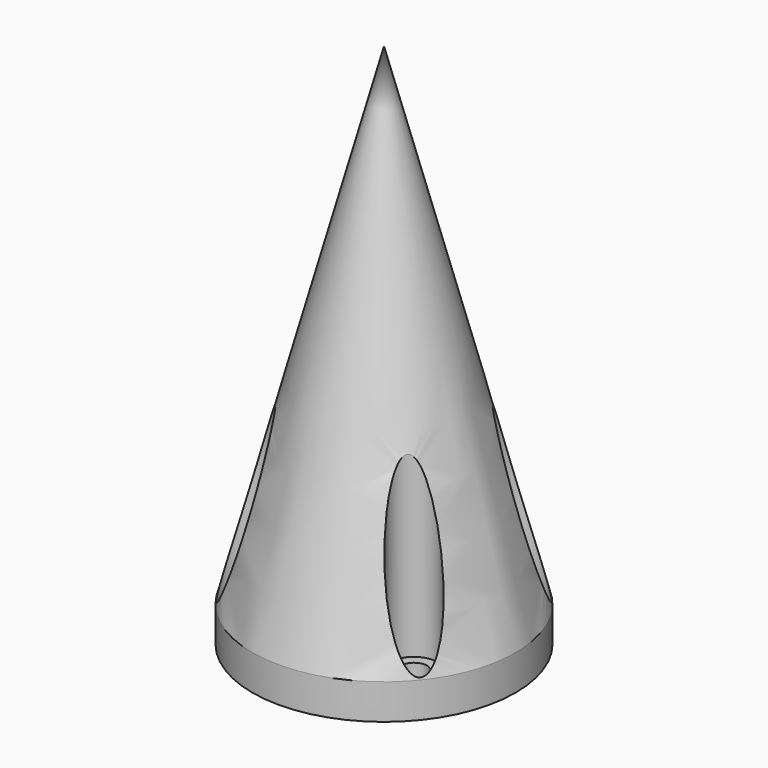
from build123d import *

# Parameters (mm, degrees)
F0_R           = 1.25
F1_DEPTH       = 5
F3_D           = 2.5
F3_DEPTH       = 5
F3_CBORE_D     = 4.4
F3_CBORE_DEPTH = 2
F3_TIP         = 0.7510757738
F4_DEPTH       = 45


# Not quite as in the source:
# - a fillet or chamfer that OpenCascade refuses, or shapes differently, is made with other operations: its cross-section is extruded or revolved along the edge and cut away or added


with BuildPart() as f1:
    # F0 (on Top) → F1 (new body)
    with BuildSketch(Plane.XY):
        with BuildLine():
            ThreePointArc((9.7397717911, -7.8349757789), (11.7897656336, -4.1534836349), (12.5, 0))
            ThreePointArc((12.5, 0), (11.7897656358, 4.1534836287), (9.7397717994, 7.8349757687))
            ThreePointArc((9.7397717994, 7.8349757687), (6.6e-09, 12.5), (-9.7397717911, 7.8349757789))
            ThreePointArc((-9.7397717911, 7.8349757789), (-12.5, 0), (-9.7397717911, -7.8349757789))
            ThreePointArc((-9.7397717911, -7.8349757789), (0, -12.5), (9.7397717911, -7.8349757789))
        make_face()
        with BuildLine():
            ThreePointArc((-5.7366128015, -6.4246802223), (-7.2389857978, -8.5468380541), (-9.7397717911, -7.8349757789))
            ThreePointArc((-9.7397717911, -7.8349757789), (-8.7342398052, -4.3025223904), (-5.7366128015, -6.4246802223))
        make_face(mode=Mode.SUBTRACT)
        with BuildLine():
            ThreePointArc((10.2366128015, -6.4246802223), (10.1087706334, -7.172307226), (9.7397717911, -7.8349757789))
            ThreePointArc((9.7397717911, -7.8349757789), (5.8644549697, -5.6770532186), (10.2366128015, -6.4246802223))
        make_face(mode=Mode.SUBTRACT)
        with BuildLine():
            ThreePointArc((-5.7366128015, 6.4246802223), (-8.7342398052, 4.3025223904), (-9.7397717911, 7.8349757789))
            ThreePointArc((-9.7397717911, 7.8349757789), (-7.2389857978, 8.5468380541), (-5.7366128015, 6.4246802223))
        make_face(mode=Mode.SUBTRACT)
        with BuildLine():
            ThreePointArc((10.2366128015, 6.4246802223), (5.8644549675, 5.6770532248), (9.7397717994, 7.8349757687))
            ThreePointArc((9.7397717994, 7.8349757687), (10.1087706356, 7.1723072198), (10.2366128015, 6.4246802223))
        make_face(mode=Mode.SUBTRACT)
        with BuildLine():
            ThreePointArc((10.2366128015, 6.4246802223), (10.1087706356, 7.1723072198), (9.7397717994, 7.8349757687))
            ThreePointArc((9.7397717994, 7.8349757687), (5.8644549675, 5.6770532248), (10.2366128015, 6.4246802223))
        make_face()
        with Locations((7.9866128015, 6.4246802223)):
            Circle(F0_R, mode=Mode.SUBTRACT)
        with BuildLine():
            ThreePointArc((10.2366128015, -6.4246802223), (5.8644549697, -5.6770532186), (9.7397717911, -7.8349757789))
            ThreePointArc((9.7397717911, -7.8349757789), (10.1087706334, -7.172307226), (10.2366128015, -6.4246802223))
        make_face()
        with Locations((7.9866128015, -6.4246802223)):
            Circle(F0_R, mode=Mode.SUBTRACT)
        with BuildLine():
            ThreePointArc((-5.7366128015, -6.4246802223), (-8.7342398052, -4.3025223904), (-9.7397717911, -7.8349757789))
            ThreePointArc((-9.7397717911, -7.8349757789), (-7.2389857978, -8.5468380541), (-5.7366128015, -6.4246802223))
        make_face()
        with Locations((-7.9866128015, -6.4246802223)):
            Circle(F0_R, mode=Mode.SUBTRACT)
        with BuildLine():
            ThreePointArc((-5.7366128015, 6.4246802223), (-7.2389857978, 8.5468380541), (-9.7397717911, 7.8349757789))
            ThreePointArc((-9.7397717911, 7.8349757789), (-8.7342398052, 4.3025223904), (-5.7366128015, 6.4246802223))
        make_face()
        with Locations((-7.9866128015, 6.4246802223)):
            Circle(F0_R, mode=Mode.SUBTRACT)
        with Locations((7.9866128015, 6.4246802223)):
            Circle(F0_R)
        with Locations((7.9866128015, -6.4246802223)):
            Circle(F0_R)
        with Locations((-7.9866128015, -6.4246802223)):
            Circle(F0_R)
        with Locations((-7.9866128015, 6.4246802223)):
            Circle(F0_R)
    extrude(amount=F1_DEPTH)

    # F3
    with Locations(Plane.XY.offset(5)):
        with Locations((-7.9866128015, 6.4246802223), (-7.9866128015, -6.4246802223), (7.9866128015, -6.4246802223), (7.9866128015, 6.4246802223)):
            CounterBoreHole(F3_D / 2, F3_CBORE_D / 2, F3_CBORE_DEPTH, depth=F3_DEPTH)
            with Locations((0, 0, -(F3_DEPTH + F3_TIP / 2))):  # 118° drill point
                Cone(0, F3_D / 2, F3_TIP, mode=Mode.SUBTRACT)

    # F4 (add): a face of the model
    f4_faces = [f1.faces().sort_by_distance(p)[0] for p in [
        (0, 0, 5),
    ]]
    extrude(f4_faces, amount=F4_DEPTH)

    # F5: chamfer of 12.5 x 46.6506350946 on 1 edges, made by hand

    # F5_s1 → F5_t2 (revolve, cut)
    with BuildSketch(Plane(origin=(0, 0, 0), x_dir=(0, 0, 1), z_dir=(0.6267980623, 0.7791817433, 0))):
        Polygon((3.3493649054, -12.5), (50, 0), (50, -12.5), align=None)
    revolve(axis=Axis((0, 0, 50), (0, 0, 1)), mode=Mode.SUBTRACT)


solid = f1.part
